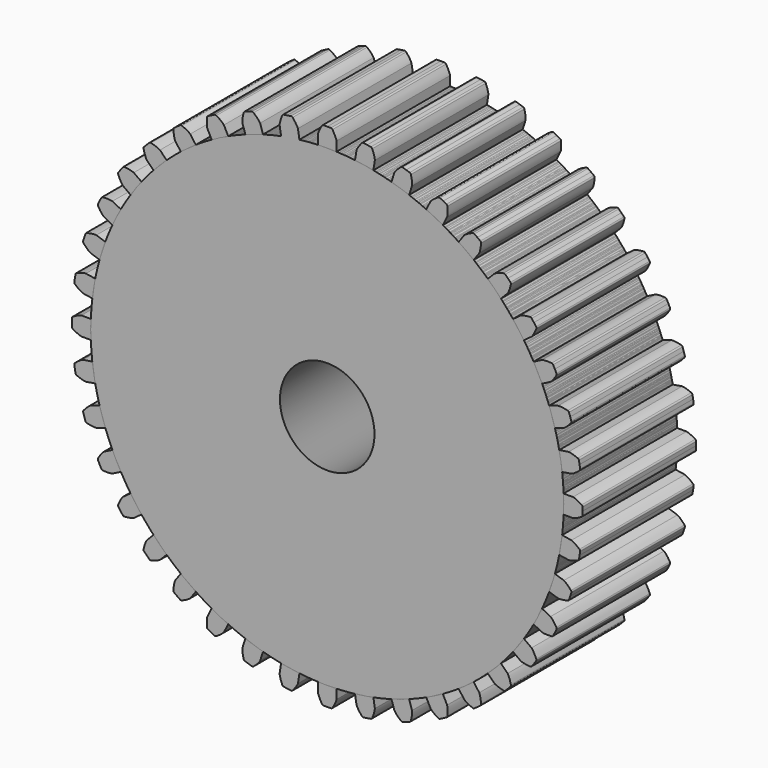
from build123d import *

# Parameters (mm, degrees)
F0_R     = 6.35
F1_DEPTH = 19.05
F2_COUNT = 40
F2_ANGLE = 351


with BuildPart() as f1:
    # F0 (on Front) → F1 (new body)
    with BuildSketch(Plane.XZ):
        with BuildLine():
            ThreePointArc((-1.2465792168, 31.7255187547), (-22.0054948804, -22.8871294632), (31.75, 0))
            ThreePointArc((31.75, 0), (22.8871294632, 22.0054948804), (1.2465792168, 31.7255187547))
            ThreePointArc((1.2465792168, 31.7255187547), (0, 31.75), (-1.2465792168, 31.7255187547))
        make_face()
        Circle(F0_R, mode=Mode.SUBTRACT)
        with BuildLine():
            ThreePointArc((-1.2465792168, 31.7255187547), (0, 31.75), (1.2465792168, 31.7255187547))
            Line((1.2465792168, 31.7255187547), (1.2465792168, 32.9955187547))
            add(Edge.make_bspline(
                [(0.70783976, 34.163171307), (0.938537613, 33.7787444715), (1.1569997034, 33.3931709244), (1.2465792168, 32.9955187547)],
                knots=[0.0488462972, 0.0488462972, 0.0488462972, 0.0488462972, 0.5145111791, 0.5145111791, 0.5145111791, 0.5145111791], degree=3))
            ThreePointArc((0.70783976, 34.163171307), (0.616771691, 34.2526011617), (0.4937040603, 34.2864456644))
            ThreePointArc((0.4937040603, 34.2864456644), (0.2468584273, 34.2891114046), (0, 34.29))
            ThreePointArc((0, 34.29), (-0.2468584273, 34.2891114046), (-0.4937040603, 34.2864456644))
            ThreePointArc((-0.4937040603, 34.2864456644), (-0.616771691, 34.2526011617), (-0.70783976, 34.163171307))
            add(Edge.make_bspline(
                [(-0.70783976, 34.163171307), (-0.938537613, 33.7787444715), (-1.1569997034, 33.3931709244), (-1.2465792168, 32.9955187547)],
                knots=[0.0488462972, 0.0488462972, 0.0488462972, 0.0488462972, 0.5145111791, 0.5145111791, 0.5145111791, 0.5145111791], degree=3))
            Line((-1.2465792168, 32.9955187547), (-1.2465792168, 31.7255187547))
        make_face()
    extrude(amount=F1_DEPTH)


with BuildPart() as f2_1:
    # F2: instance of F1
    add(f1.part.rotate(Axis((0, 0, 0), (0, 1, 0)), 1 * F2_ANGLE / (F2_COUNT - 1)))


with BuildPart() as f2_2:
    # F2: instance of F1
    add(f1.part.rotate(Axis((0, 0, 0), (0, 1, 0)), 2 * F2_ANGLE / (F2_COUNT - 1)))


with BuildPart() as f2_3:
    # F2: instance of F1
    add(f1.part.rotate(Axis((0, 0, 0), (0, 1, 0)), 3 * F2_ANGLE / (F2_COUNT - 1)))


with BuildPart() as f2_4:
    # F2: instance of F1
    add(f1.part.rotate(Axis((0, 0, 0), (0, 1, 0)), 4 * F2_ANGLE / (F2_COUNT - 1)))


with BuildPart() as f2_5:
    # F2: instance of F1
    add(f1.part.rotate(Axis((0, 0, 0), (0, 1, 0)), 5 * F2_ANGLE / (F2_COUNT - 1)))


with BuildPart() as f2_6:
    # F2: instance of F1
    add(f1.part.rotate(Axis((0, 0, 0), (0, 1, 0)), 6 * F2_ANGLE / (F2_COUNT - 1)))


with BuildPart() as f2_7:
    # F2: instance of F1
    add(f1.part.rotate(Axis((0, 0, 0), (0, 1, 0)), 7 * F2_ANGLE / (F2_COUNT - 1)))


with BuildPart() as f2_8:
    # F2: instance of F1
    add(f1.part.rotate(Axis((0, 0, 0), (0, 1, 0)), 8 * F2_ANGLE / (F2_COUNT - 1)))


with BuildPart() as f2_9:
    # F2: instance of F1
    add(f1.part.rotate(Axis((0, 0, 0), (0, 1, 0)), 9 * F2_ANGLE / (F2_COUNT - 1)))


with BuildPart() as f2_10:
    # F2: instance of F1
    add(f1.part.rotate(Axis((0, 0, 0), (0, 1, 0)), 10 * F2_ANGLE / (F2_COUNT - 1)))


with BuildPart() as f2_11:
    # F2: instance of F1
    add(f1.part.rotate(Axis((0, 0, 0), (0, 1, 0)), 11 * F2_ANGLE / (F2_COUNT - 1)))


with BuildPart() as f2_12:
    # F2: instance of F1
    add(f1.part.rotate(Axis((0, 0, 0), (0, 1, 0)), 12 * F2_ANGLE / (F2_COUNT - 1)))


with BuildPart() as f2_13:
    # F2: instance of F1
    add(f1.part.rotate(Axis((0, 0, 0), (0, 1, 0)), 13 * F2_ANGLE / (F2_COUNT - 1)))


with BuildPart() as f2_14:
    # F2: instance of F1
    add(f1.part.rotate(Axis((0, 0, 0), (0, 1, 0)), 14 * F2_ANGLE / (F2_COUNT - 1)))


with BuildPart() as f2_15:
    # F2: instance of F1
    add(f1.part.rotate(Axis((0, 0, 0), (0, 1, 0)), 15 * F2_ANGLE / (F2_COUNT - 1)))


with BuildPart() as f2_16:
    # F2: instance of F1
    add(f1.part.rotate(Axis((0, 0, 0), (0, 1, 0)), 16 * F2_ANGLE / (F2_COUNT - 1)))


with BuildPart() as f2_17:
    # F2: instance of F1
    add(f1.part.rotate(Axis((0, 0, 0), (0, 1, 0)), 17 * F2_ANGLE / (F2_COUNT - 1)))


with BuildPart() as f2_18:
    # F2: instance of F1
    add(f1.part.rotate(Axis((0, 0, 0), (0, 1, 0)), 18 * F2_ANGLE / (F2_COUNT - 1)))


with BuildPart() as f2_19:
    # F2: instance of F1
    add(f1.part.rotate(Axis((0, 0, 0), (0, 1, 0)), 19 * F2_ANGLE / (F2_COUNT - 1)))


with BuildPart() as f2_20:
    # F2: instance of F1
    add(f1.part.rotate(Axis((0, 0, 0), (0, 1, 0)), 20 * F2_ANGLE / (F2_COUNT - 1)))


with BuildPart() as f2_21:
    # F2: instance of F1
    add(f1.part.rotate(Axis((0, 0, 0), (0, 1, 0)), 21 * F2_ANGLE / (F2_COUNT - 1)))


with BuildPart() as f2_22:
    # F2: instance of F1
    add(f1.part.rotate(Axis((0, 0, 0), (0, 1, 0)), 22 * F2_ANGLE / (F2_COUNT - 1)))


with BuildPart() as f2_23:
    # F2: instance of F1
    add(f1.part.rotate(Axis((0, 0, 0), (0, 1, 0)), 23 * F2_ANGLE / (F2_COUNT - 1)))


with BuildPart() as f2_24:
    # F2: instance of F1
    add(f1.part.rotate(Axis((0, 0, 0), (0, 1, 0)), 24 * F2_ANGLE / (F2_COUNT - 1)))


with BuildPart() as f2_25:
    # F2: instance of F1
    add(f1.part.rotate(Axis((0, 0, 0), (0, 1, 0)), 25 * F2_ANGLE / (F2_COUNT - 1)))


with BuildPart() as f2_26:
    # F2: instance of F1
    add(f1.part.rotate(Axis((0, 0, 0), (0, 1, 0)), 26 * F2_ANGLE / (F2_COUNT - 1)))


with BuildPart() as f2_27:
    # F2: instance of F1
    add(f1.part.rotate(Axis((0, 0, 0), (0, 1, 0)), 27 * F2_ANGLE / (F2_COUNT - 1)))


with BuildPart() as f2_28:
    # F2: instance of F1
    add(f1.part.rotate(Axis((0, 0, 0), (0, 1, 0)), 28 * F2_ANGLE / (F2_COUNT - 1)))


with BuildPart() as f2_29:
    # F2: instance of F1
    add(f1.part.rotate(Axis((0, 0, 0), (0, 1, 0)), 29 * F2_ANGLE / (F2_COUNT - 1)))


with BuildPart() as f2_30:
    # F2: instance of F1
    add(f1.part.rotate(Axis((0, 0, 0), (0, 1, 0)), 30 * F2_ANGLE / (F2_COUNT - 1)))


with BuildPart() as f2_31:
    # F2: instance of F1
    add(f1.part.rotate(Axis((0, 0, 0), (0, 1, 0)), 31 * F2_ANGLE / (F2_COUNT - 1)))


with BuildPart() as f2_32:
    # F2: instance of F1
    add(f1.part.rotate(Axis((0, 0, 0), (0, 1, 0)), 32 * F2_ANGLE / (F2_COUNT - 1)))


with BuildPart() as f2_33:
    # F2: instance of F1
    add(f1.part.rotate(Axis((0, 0, 0), (0, 1, 0)), 33 * F2_ANGLE / (F2_COUNT - 1)))


with BuildPart() as f2_34:
    # F2: instance of F1
    add(f1.part.rotate(Axis((0, 0, 0), (0, 1, 0)), 34 * F2_ANGLE / (F2_COUNT - 1)))


with BuildPart() as f2_35:
    # F2: instance of F1
    add(f1.part.rotate(Axis((0, 0, 0), (0, 1, 0)), 35 * F2_ANGLE / (F2_COUNT - 1)))


with BuildPart() as f2_36:
    # F2: instance of F1
    add(f1.part.rotate(Axis((0, 0, 0), (0, 1, 0)), 36 * F2_ANGLE / (F2_COUNT - 1)))


with BuildPart() as f2_37:
    # F2: instance of F1
    add(f1.part.rotate(Axis((0, 0, 0), (0, 1, 0)), 37 * F2_ANGLE / (F2_COUNT - 1)))


with BuildPart() as f2_38:
    # F2: instance of F1
    add(f1.part.rotate(Axis((0, 0, 0), (0, 1, 0)), 38 * F2_ANGLE / (F2_COUNT - 1)))


with BuildPart() as f2_39:
    # F2: instance of F1
    add(f1.part.rotate(Axis((0, 0, 0), (0, 1, 0)), 39 * F2_ANGLE / (F2_COUNT - 1)))


solid = Compound([f1.part, f2_1.part, f2_2.part, f2_3.part, f2_4.part, f2_5.part, f2_6.part, f2_7.part, f2_8.part, f2_9.part, f2_10.part, f2_11.part, f2_12.part, f2_13.part, f2_14.part, f2_15.part, f2_16.part, f2_17.part, f2_18.part, f2_19.part, f2_20.part, f2_21.part, f2_22.part, f2_23.part, f2_24.part, f2_25.part, f2_26.part, f2_27.part, f2_28.part, f2_29.part, f2_30.part, f2_31.part, f2_32.part, f2_33.part, f2_34.part, f2_35.part, f2_36.part, f2_37.part, f2_38.part, f2_39.part])
